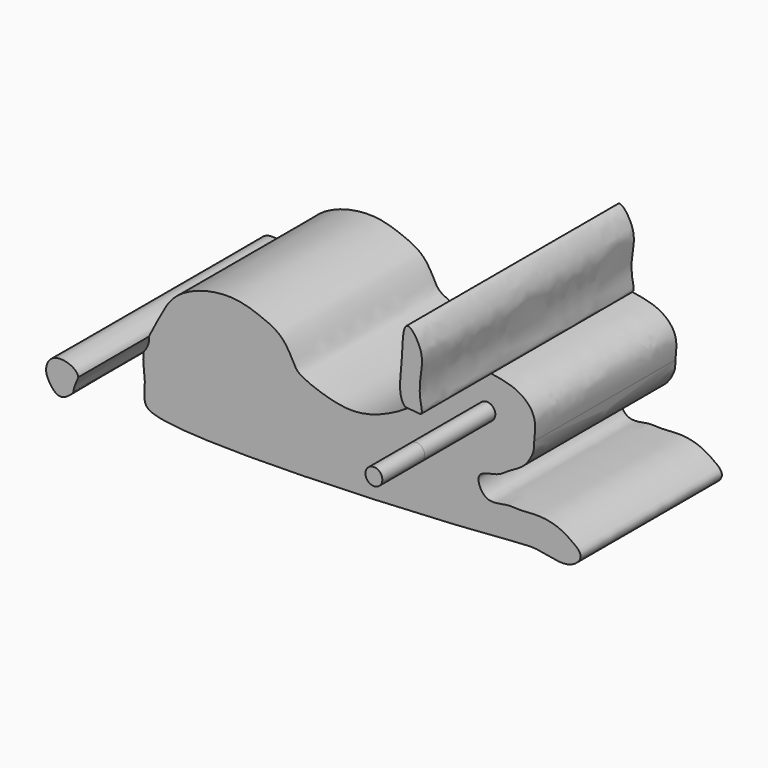
from build123d import *

# Parameters (mm, degrees)
F1_DEPTH = 76.2
F2_R     = 2.4319130927
F3_DEPTH = 12.7
F4_DEPTH = 2.54
F5_DEPTH = 25.4


with BuildPart() as f1:
    # F0 (on Front) → F1 (new body)
    with BuildSketch(Plane.XZ):
        with BuildLine():
            add(Edge.make_bspline(
                [(44.5040464401, 26.9942544401), (43.7025207143, 26.2449339369), (41.3940822523, 26.3468172293), (40.1204258352, 27.4624891095)],
                knots=[0.8919576844, 0.8919576844, 0.8919576844, 0.8919576844, 1, 1, 1, 1], degree=3))
            add(Edge.make_bspline(
                [(40.1204258352, 27.4624891095), (38.9360947969, 27.5086026747), (35.5507022413, 27.3547831172), (30.715316621, 24.5145429625), (27.549615074, 16.7800645689), (21.3367269152, 10.1778572579), (9.690225897, 4.5337814089), (0.4909328579, 4.3226200092), (-10.5226815139, 8.3297199529), (-12.2049833552, 10.8074582653), (-15.1070696494, 17.1143533318), (-21.9457581229, 20.0782616448), (-29.1520626347, 22.4927855247), (-38.8059668984, 21.5103761789), (-47.4246645535, 17.1084565784), (-50.5371723174, 10.8344917909), (-53.1588308159, 6.0932356033), (-53.9547677358, 4.3626299569)],
                knots=[0.0920177892, 0.0920177892, 0.0920177892, 0.0920177892, 0.1044306128, 0.1287974644, 0.1563855317, 0.1858969699, 0.220317271, 0.2508080941, 0.2829987651, 0.2997255812, 0.3243405086, 0.3507495419, 0.3776085905, 0.4077900186, 0.4373433756, 0.4657256658, 0.4824978765, 0.4824978765, 0.4824978765, 0.4824978765], degree=3))
            add(Edge.make_bspline(
                [(-55.4476603866, 0), (-54.3323025136, 1.35837208), (-53.6778969091, 3.0660661447), (-53.9547677358, 4.3626299569)],
                knots=[0.8473848473, 0.8473848473, 0.8473848473, 0.8473848473, 1, 1, 1, 1], degree=3))
            add(Edge.make_bspline(
                [(-55.4476603866, 0), (-55.8367791323, -2.2336624741), (-54.8979671013, -5.8743579042), (-55.3649348107, -11.5763798366), (-54.2676743855, -19.4792978799), (47.893929392, -14.3433493463), (57.0984201671, -12.5503749206), (66.7585309989, -15.5153831326), (71.6413073611, -10.8813936834), (67.651608515, -7.7901322668), (63.6434344788, -5.2720688424), (57.894437502, -4.3371630294), (53.2310787605, -5.091559031), (48.9673008094, -4.4181140537), (42.5640373489, -6.6215596861), (39.3614174037, 1.2522575321), (46.4581410781, 1.4638363333), (49.6896797698, 4.3220120909), (54.2947853073, 6.2613734221), (57.0400872236, 11.1920257082), (56.8381486744, 12.8225743471), (56.906811893, 13.8619150966)],
                knots=[0.497166276, 0.497166276, 0.497166276, 0.497166276, 0.5212772581, 0.5438863274, 0.5642256362, 0.6611142266, 0.6962188111, 0.7243801021, 0.7454491245, 0.764500156, 0.7863733796, 0.8096634303, 0.8306890319, 0.851139695, 0.8747541093, 0.897125901, 0.9194976922, 0.9401504965, 0.9618408842, 0.9839800429, 1, 1, 1, 1], degree=3))
            add(Edge.make_bspline(
                [(56.906811893, 13.8619150966), (57.0080256879, 15.3939670994), (57.9092168831, 20.1692609502), (52.7545495628, 25.6517146313), (47.3263555943, 26.5820452218), (44.5040464401, 26.9942544401)],
                knots=[0, 0, 0, 0, 0.0236143992, 0.0489649056, 0.0771563834, 0.0771563834, 0.0771563834, 0.0771563834], degree=3))
        make_face()
    extrude(amount=F1_DEPTH)

    # F2 (on face) → F3 (join)
    with BuildSketch(Plane.XZ.offset(76.2)):
        with Locations((43.2880856097, 17.0234050602)):
            Circle(F2_R)
    extrude(amount=F3_DEPTH)

    # F4 (add): a face of the model
    f4_faces = [f1.faces().sort_by_distance(p)[0] for p in [
        (43.2880856097, -88.9, 17.0234050602),
    ]]
    extrude(f4_faces, amount=F4_DEPTH)

    # F5 (cut): a face of the model
    f5_faces = [f1.faces().sort_by_distance(p)[0] for p in [
        (2.0508288129, -76.2, 0.9168755014),
    ]]
    extrude(f5_faces, amount=-F5_DEPTH, mode=Mode.SUBTRACT)


with BuildPart() as f1b:
    # F0 (on Front) → F1, piece 2 (new body)
    with BuildSketch(Plane.XZ):
        with BuildLine():
            add(Edge.make_bspline(
                [(40.1204258352, 27.4624891095), (38.573237263, 28.8177641745), (38.5334436907, 34.4298351403), (39.2933915498, 38.9020936), (39.3666336438, 51.8061735204), (45.8289660834, 42.7639227626), (44.2908641443, 36.6648823613), (44.1351473438, 30.7270519338), (45.2084271192, 27.6527571778), (44.5040464401, 26.9942544401)],
                knots=[0, 0, 0, 0, 0.1312456278, 0.2583271636, 0.407431011, 0.5358549223, 0.670131063, 0.7970101148, 0.8919576844, 0.8919576844, 0.8919576844, 0.8919576844], degree=3))
            add(Edge.make_bspline(
                [(44.5040464401, 26.9942544401), (43.0162393027, 27.2115544535), (41.5383807527, 27.4072790758), (40.1204258352, 27.4624891095)],
                knots=[0.0771563834, 0.0771563834, 0.0771563834, 0.0771563834, 0.0920177892, 0.0920177892, 0.0920177892, 0.0920177892], degree=3))
        make_face()
    extrude(amount=F1_DEPTH)


with BuildPart() as f1c:
    # F0 (on Front) → F1, piece 3 (new body)
    with BuildSketch(Plane.XZ):
        with BuildLine():
            add(Edge.make_bspline(
                [(-53.9547677358, 4.3626299569), (-54.6508668327, 2.8491016892), (-55.2109321947, 1.3588933568), (-55.4476603866, 0)],
                knots=[0.4824978765, 0.4824978765, 0.4824978765, 0.4824978765, 0.497166276, 0.497166276, 0.497166276, 0.497166276], degree=3))
            add(Edge.make_bspline(
                [(-53.9547677358, 4.3626299569), (-54.1950769782, 5.487978811), (-56.2514707817, 7.2687545626), (-61.7294511282, 7.7201431922), (-63.841342532, 3.3153788735), (-62.2023861696, -0.0071278235), (-59.4472931082, -3.2134699608), (-56.5451452134, -1.3366048541), (-55.4476603866, 0)],
                knots=[0, 0, 0, 0, 0.1324618855, 0.2892053657, 0.429945451, 0.5650819103, 0.6972152752, 0.8473848473, 0.8473848473, 0.8473848473, 0.8473848473], degree=3))
        make_face()
    extrude(amount=F1_DEPTH)


solid = Compound([f1.part, f1b.part, f1c.part])
